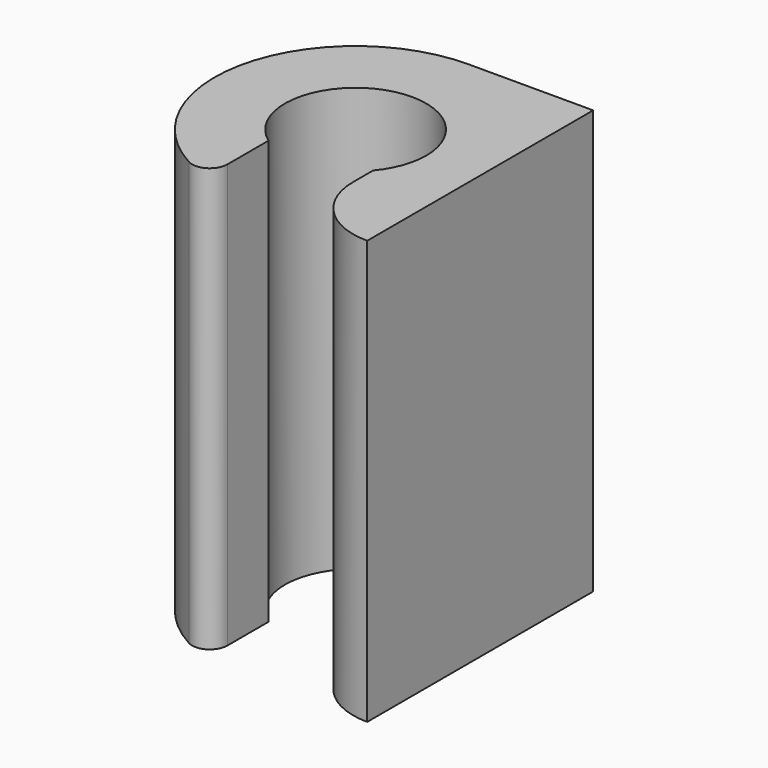
from build123d import *

# Parameters (mm, degrees)
F1_DEPTH = 12
F2_R     = 1.99999


# Not quite as in the source:
# - a fillet or chamfer is up to 0.001 mm smaller than in the source, because OpenCascade refuses the exact size
# - a feature names something its author has since deleted; it is built from what else it names


with BuildPart() as f1:
    # F0 (on Top) → F1 (new body)
    with BuildSketch(Plane.XY):
        with BuildLine():
            Line((2, 14.3612188522), (0, 14.3612188522))
            Line((0, 14.3612188522), (0, 11.6508584444))
            ThreePointArc((0, 11.6508584444), (0.4713307349, 10.3612188522), (0, 9.0715792599))
            Line((0, 9.0715792599), (0, 6.3612188522))
            Line((0, 6.3612188522), (2, 6.3612188522))
            Line((2, 6.3612188522), (2, 14.3612188522))
        make_face()
        with BuildLine():
            Line((0, 11.6508584444), (0, 14.3612188522))
            Line((0, 14.3612188522), (-1.5286692651, 14.3612188522))
            ThreePointArc((-1.5286692651, 14.3612188522), (-5.4053887158, 11.346635668), (-3.4387615336, 6.8467420026))
            ThreePointArc((-3.4387615336, 6.8467420026), (-2.9444425376, 6.8562954182), (-2.7, 7.2860516088))
            Line((-2.7, 7.2860516088), (-2.7, 8.7401129613))
            ThreePointArc((-2.7, 8.7401129613), (-2.9949681852, 11.7213539472), (0, 11.6508584444))
        make_face()
    extrude(amount=F1_DEPTH)

    # F2 (radius 2 in the source; OpenCascade refuses exactly that, so slightly less here)
    f2_edges = [f1.edges().sort_by_distance(p)[0] for p in [
        (0, 6.361219, 6),
    ]]
    fillet(f2_edges, radius=F2_R)


solid = f1.part
